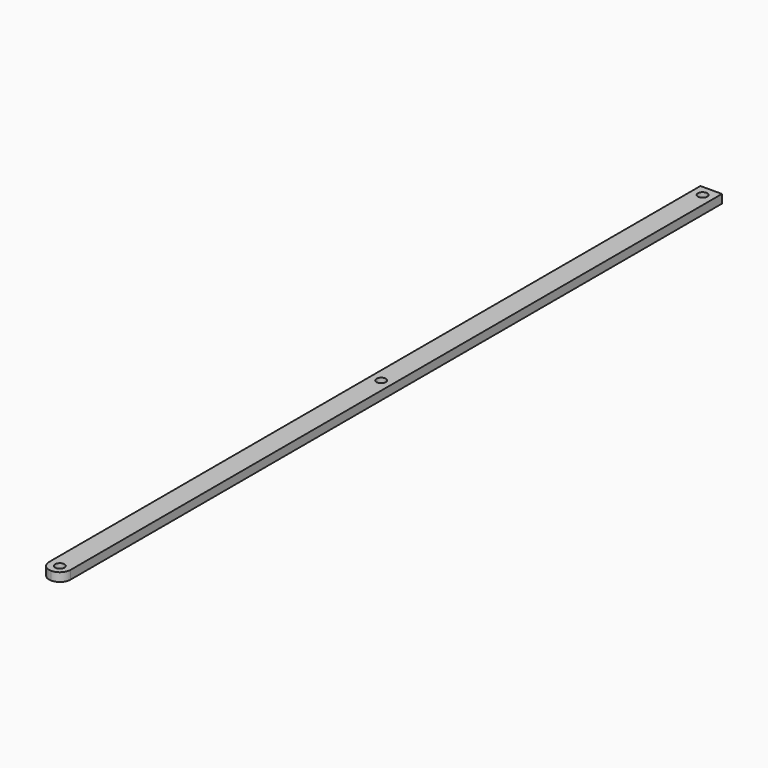
from build123d import *

# Parameters (mm, degrees)
F0_W     = 7.9375
F0_H     = 304.8
F0_R     = 1.7272
F1_DEPTH = 3.175
F2_R     = 1.7272
F3_DEPTH = 3.175
F4_R     = 3.96874


# Not quite as in the source:
# - a fillet or chamfer is up to 0.001 mm smaller than in the source, because OpenCascade refuses the exact size


with BuildPart() as f1:
    # F0 (on Top) → F1 (new body)
    with BuildSketch(Plane.XY):
        Rectangle(F0_W, F0_H)
        Circle(F0_R, mode=Mode.SUBTRACT)
    extrude(amount=F1_DEPTH)

    # F2 (on face) → F3 (cut, through all)
    with BuildSketch(Plane.XY.offset(3.175)):
        with Locations((0, 148.43125)):
            Circle(F2_R)
        with Locations((0, -148.43125)):
            Circle(F2_R)
    extrude(amount=-F3_DEPTH, mode=Mode.SUBTRACT)

    # F4 (radius 3.96875 in the source; OpenCascade refuses exactly that, so slightly less here)
    f4_edges = [f1.edges().sort_by_distance(p)[0] for p in [
        (-3.96875, -152.4, 1.5875),
        (3.96875, -152.4, 1.5875),
    ]]
    fillet(f4_edges, radius=F4_R)


solid = f1.part
